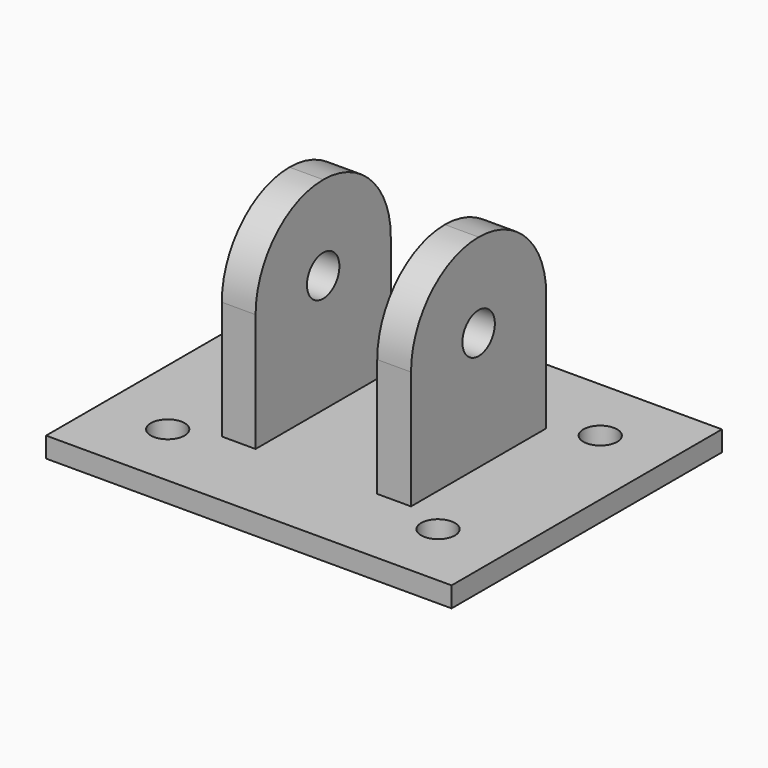
from build123d import *

# Parameters (mm, degrees)
F0_W     = 60
F0_H     = 50
F1_DEPTH = 3
F2_W     = 5
F2_H     = 25
F3_DEPTH = 30
F4_R     = 12.49999
F5_R     = 3
F6_DEPTH = 50
F7_R     = 2.5
F8_DEPTH = 25


# Not quite as in the source:
# - a fillet or chamfer is up to 0.001 mm smaller than in the source, because OpenCascade refuses the exact size


with BuildPart() as f1:
    # F0 (on Top) → F1 (new body)
    with BuildSketch(Plane.XY):
        Rectangle(F0_W, F0_H)
    extrude(amount=F1_DEPTH)

    # F2 (on face) → F3 (join)
    with BuildSketch(Plane.XY.offset(3)):
        with Locations((-11.5, 0)):
            Rectangle(F2_W, F2_H)
        with Locations((11.5, 0)):
            Rectangle(F2_W, F2_H)
    extrude(amount=F3_DEPTH)

    # F4 (radius 12.5 in the source; OpenCascade refuses exactly that, so slightly less here)
    f4_edges = [f1.edges().sort_by_distance(p)[0] for p in [
        (-11.5, -12.5, 33),
        (-11.5, 12.5, 33),
        (11.5, 12.5, 33),
        (11.5, -12.5, 33),
    ]]
    fillet(f4_edges, radius=F4_R)

    # F5 (on face) → F6 (cut)
    with BuildSketch(Plane(origin=(-14, 0, 0), x_dir=(0, -1, 0), z_dir=(-1, 0, 0))):
        with Locations((0, 20.5)):
            Circle(F5_R)
    extrude(amount=-F6_DEPTH, mode=Mode.SUBTRACT)

    # F7 (on face) → F8 (cut)
    with BuildSketch(Plane.XY.offset(3)):
        with Locations((-20, -15)):
            Circle(F7_R)
        with Locations((-20, 15)):
            Circle(F7_R)
        with Locations((20, 15)):
            Circle(F7_R)
        with Locations((20, -15)):
            Circle(F7_R)
    extrude(amount=-F8_DEPTH, mode=Mode.SUBTRACT)


solid = f1.part
